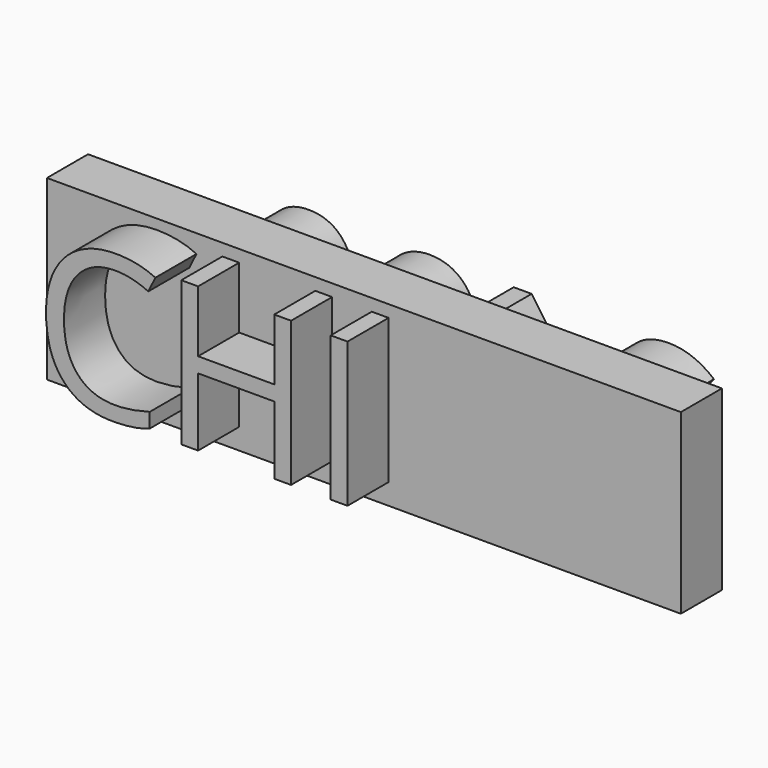
from build123d import *

# Parameters (mm, degrees)
F1_TEXT_SIZE = 39.4314501642
F2_DEPTH     = 20
F0_W         = 123.42556566
F0_H         = 34.5665328205
F3_DEPTH     = 10
F4_TEXT_SIZE = 40.643918328
F5_DEPTH     = 10


# Not quite as in the source:
# - Text() gives the source's letters only with a copy of the font that has no kerning and outlines rounded to 1/6400 em; it was checked with that copy


with BuildPart() as f2:
    # F1 (on face) → F2 (new body)
    with BuildSketch(Plane.XZ):
        with Locations((5.4098321125, 4.065496847)):
            Text('CHI', F1_TEXT_SIZE, font='Open Sans', text_align=(TextAlign.LEFT, TextAlign.BOTTOM))
    extrude(amount=F2_DEPTH)


with BuildPart() as f3:
    # F0 (on Front) → F3 (new body)
    with BuildSketch(Plane.XZ):
        with Locations((61.71278283, 17.2832664102)):
            Rectangle(F0_W, F0_H)
    extrude(amount=F3_DEPTH)


with BuildPart() as f5:
    # F4 (on face) → F5 (new body)
    with BuildSketch(Plane(origin=(0, 0, 0), x_dir=(-1, 0, 0), z_dir=(0, 1, 0))):
        with Locations((-116.240285337, 2.883868292)):
            Text('2490', F4_TEXT_SIZE, font='Open Sans', text_align=(TextAlign.LEFT, TextAlign.BOTTOM))
    extrude(amount=F5_DEPTH)


solid = Compound([f2.part, f3.part, f5.part])
